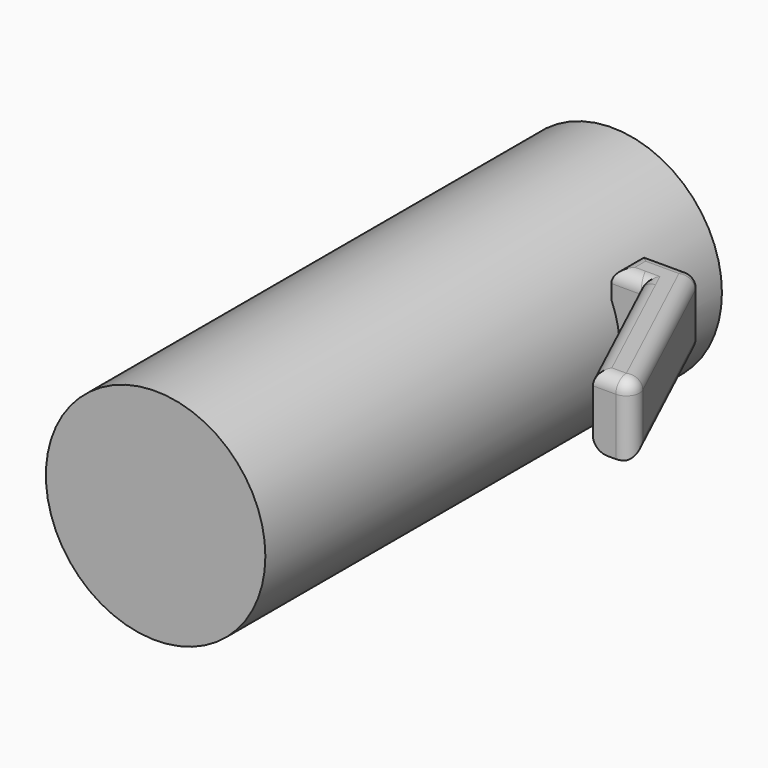
from build123d import *

# Parameters (mm, degrees)
F0_R          = 31.75
F0_R_2        = 28.575
F1_DEPTH      = 165.1
F3_DEPTH      = 20.32
F4_T1_DEPTH   = 16.51
F4_T3_DEPTH   = 12.7
F4_T5_DEPTH   = 50.1912424643
F4_T7_DEPTH   = 13.4477623063
F4_T9_DEPTH   = 11.43
F4_T14_DEPTH  = 3.8862
F4_T20_DEPTH  = 3.8862
F4_T26_DEPTH  = 3.8862
F4_T32_DEPTH  = 65.6967445131
F4_T37_DEPTH  = 18.118286919
F4_T42_DEPTH  = 65.037372593
F4_T48_DEPTH  = 16.1561075649
F4_T53_DEPTH  = 65.037372593
F4_T59_DEPTH  = 20.4327623063
F4_S60_R      = 31.75
F4_T61_DEPTH  = 12
F4_T66_DEPTH  = 65.6967445131
F4_T70_DEPTH  = 31.461255122
F4_T77_DEPTH  = 20.955
F4_T81_DEPTH  = 22.9727623063
F4_T88_DEPTH  = 27.643286919
F4_T92_DEPTH  = 20.955
F4_T99_DEPTH  = 18.118286919
F4_T103_DEPTH = 65.037372593
F4_T110_DEPTH = 16.1561075649
F4_T114_DEPTH = 65.037372593
F5_R          = 27.6352
F6_DEPTH      = 161.925


# Not quite as in the source:
# - a fillet or chamfer that OpenCascade refuses, or shapes differently, is made with other operations: its cross-section is extruded or revolved along the edge and cut away or added


with BuildPart() as f1:
    # F0 (on Front) → F1 (new body)
    with BuildSketch(Plane.XZ):
        Circle(F0_R)
        Circle(F0_R_2, mode=Mode.SUBTRACT)
        Circle(F0_R_2)
    extrude(amount=F1_DEPTH)

    # F2 (on Top) → F3 (join)
    with BuildSketch(Plane.XY):
        Polygon((45.085, -25.4), (29.21, -25.4), (29.21, -36.83), (37.803286919, -36.83), (57.2383903863, -78.5087138864), (69.85, -78.5087138864), align=None)
    extrude(amount=F3_DEPTH)

    # F4: fillet of radius 3.81 on 11 edges, made by hand

    # F4_s2 → F4_t1 (cut)
    with BuildSketch(Plane.XY):
        with BuildLine():
            ThreePointArc((67.3225306198, -73.0885383092), (67.0828193597, -76.7458253942), (63.8694979512, -78.5087138864))
            Line((63.8694979512, -78.5087138864), (63.8694979512, -78.5849138864))
            Line((63.8694979512, -78.5849138864), (69.969610041, -78.5849138864))
            Line((69.969610041, -78.5849138864), (67.3915912732, -73.0563347976))
            Line((67.3915912732, -73.0563347976), (67.3225306198, -73.0885383092))
        make_face()
    extrude(amount=F4_T1_DEPTH, mode=Mode.SUBTRACT)

    # F4_s4 → F4_t3 (cut)
    with BuildSketch(Plane.XY.offset(3.81)):
        with BuildLine():
            ThreePointArc((42.6577623063, -25.4), (44.7048738141, -25.9966785915), (46.1107949749, -27.5998244228))
            Line((46.1107949749, -27.5998244228), (46.1798556283, -27.5676209112))
            Line((46.1798556283, -27.5676209112), (45.1335447539, -25.3238))
            Line((45.1335447539, -25.3238), (42.6577623063, -25.3238))
            Line((42.6577623063, -25.3238), (42.6577623063, -25.4))
        make_face()
    extrude(amount=F4_T3_DEPTH, mode=Mode.SUBTRACT)

    # F4_s6 → F4_t5 (cut)
    with BuildSketch(Plane(origin=(40.018755356, -85.8204978112, 0), x_dir=(0, 0, 1), z_dir=(-0.4226182617, 0.906307787, 0))):
        with BuildLine():
            ThreePointArc((16.51, 30.1263827303), (19.2040768363, 29.0104595667), (20.32, 26.3163827303))
            Line((20.32, 26.3163827303), (20.3962, 26.3163827303))
            Line((20.3962, 26.3163827303), (20.3962, 30.2025827303))
            Line((20.3962, 30.2025827303), (16.51, 30.2025827303))
            Line((16.51, 30.2025827303), (16.51, 30.1263827303))
        make_face()
    extrude(amount=F4_T5_DEPTH, mode=Mode.SUBTRACT)

    # F4_s8 → F4_t7 (cut)
    with BuildSketch(Plane.YZ.offset(29.21)):
        with BuildLine():
            ThreePointArc((-25.4, 16.51), (-26.5159231637, 19.2040768363), (-29.21, 20.32))
            Line((-29.21, 20.32), (-29.21, 20.3962))
            Line((-29.21, 20.3962), (-25.3238, 20.3962))
            Line((-25.3238, 20.3962), (-25.3238, 16.51))
            Line((-25.3238, 16.51), (-25.4, 16.51))
        make_face()
    extrude(amount=F4_T7_DEPTH, mode=Mode.SUBTRACT)

    # F4_s10 → F4_t9 (cut)
    with BuildSketch(Plane.XZ.offset(25.4)):
        with BuildLine():
            ThreePointArc((29.21, 16.51), (30.3259231637, 19.2040768363), (33.02, 20.32))
            Line((33.02, 20.32), (33.02, 20.3962))
            Line((33.02, 20.3962), (29.1338, 20.3962))
            Line((29.1338, 20.3962), (29.1338, 16.51))
            Line((29.1338, 16.51), (29.21, 16.51))
        make_face()
    extrude(amount=F4_T9_DEPTH, mode=Mode.SUBTRACT)


with BuildPart() as f4_tool12:
    # F4_s13 → F4_t14 (new body)
    with BuildSketch(Plane.XY.offset(16.51)):
        Polygon((63.8694979512, -74.6987138864), (67.3915912732, -73.0563347976), (69.969610041, -78.5849138864), (63.8694979512, -78.5849138864), align=None)
    extrude(amount=F4_T14_DEPTH)

    # F4_s15 → F4_t16 (revolve, cut)
    with BuildSketch(Plane(origin=(63.8694979512, -74.6987138864, 16.51), x_dir=(-0.8433914458, 0.5372996083, 0), z_dir=(0.5372996083, 0.8433914458, 0))):
        with BuildLine():
            ThreePointArc((0, -3.81), (3.81, 0), (0, 3.81))
            Line((0, 3.81), (0, -3.81))
        make_face()
    revolve(axis=Axis((63.8694979512, -74.6987138864, 16.51), (0, 0, 1)), mode=Mode.SUBTRACT)


with BuildPart() as f1_1:
    add(f1.part)

    # F4_t11: cut F4_tool12
    add(f4_tool12.part, mode=Mode.SUBTRACT)


with BuildPart() as f4_tool18:
    # F4_s19 → F4_t20 (new body)
    with BuildSketch(Plane.XY.offset(3.81)):
        Polygon((42.6577623063, -29.21), (42.6577623063, -25.3238), (45.1335447539, -25.3238), (46.1798556283, -27.5676209112), align=None)
    extrude(amount=-F4_T20_DEPTH)

    # F4_s21 → F4_t22 (revolve, cut)
    with BuildSketch(Plane(origin=(42.6577623063, -29.21, 3.81), x_dir=(-0.5372996083, -0.8433914458, 0), z_dir=(0.8433914458, -0.5372996083, 0))):
        with BuildLine():
            ThreePointArc((0, -3.81), (3.81, 0), (0, 3.81))
            Line((0, 3.81), (0, -3.81))
        make_face()
    revolve(axis=Axis((42.6577623063, -29.21, 3.81), (0, 0, -1)), mode=Mode.SUBTRACT)


with BuildPart() as f1_2:
    add(f1_1.part)

    # F4_t17: cut F4_tool18
    add(f4_tool18.part, mode=Mode.SUBTRACT)


with BuildPart() as f4_tool24:
    # F4_s25 → F4_t26 (new body)
    with BuildSketch(Plane.XY.offset(16.51)):
        Polygon((42.6577623063, -29.21), (42.6577623063, -25.3238), (45.1335447539, -25.3238), (46.1798556283, -27.5676209112), align=None)
    extrude(amount=F4_T26_DEPTH)

    # F4_s27 → F4_t28 (revolve, cut)
    with BuildSketch(Plane(origin=(42.6577623063, -29.21, 16.51), x_dir=(-0.5372996083, -0.8433914458, 0), z_dir=(-0.8433914458, 0.5372996083, 0))):
        with BuildLine():
            ThreePointArc((0, -3.81), (3.81, 0), (0, 3.81))
            Line((0, 3.81), (0, -3.81))
        make_face()
    revolve(axis=Axis((42.6577623063, -29.21, 16.51), (0, 0, 1)), mode=Mode.SUBTRACT)


with BuildPart() as f1_3:
    add(f1_2.part)

    # F4_t23: cut F4_tool24
    add(f4_tool24.part, mode=Mode.SUBTRACT)


with BuildPart() as f4_tool30:
    # F4_s31 → F4_t32 (new body)
    with BuildSketch(Plane(origin=(46.5716636793, -99.87325506, 0), x_dir=(0, 0, 1), z_dir=(-0.4226182617, 0.906307787, 0))):
        with BuildLine():
            ThreePointArc((0, 26.3163827303), (1.1159231637, 29.0104595667), (3.81, 30.1263827303))
            Line((3.81, 30.1263827303), (3.81, 30.2025827303))
            Line((3.81, 30.2025827303), (-0.0762, 30.2025827303))
            Line((-0.0762, 30.2025827303), (-0.0762, 26.3163827303))
            Line((-0.0762, 26.3163827303), (0, 26.3163827303))
        make_face()
    extrude(amount=F4_T32_DEPTH)

    split(bisect_by=Plane.XZ.offset(78.5087138864), keep=Keep.BOTTOM)


with BuildPart() as f1_4:
    add(f1_3.part)

    # F4_t29: cut F4_tool30
    add(f4_tool30.part, mode=Mode.SUBTRACT)


with BuildPart() as f4_tool35:
    # F4_s36 → F4_t37 (new body)
    with BuildSketch(Plane.YZ.offset(29.21)):
        with BuildLine():
            ThreePointArc((-36.83, 16.51), (-35.7140768363, 19.2040768363), (-33.02, 20.32))
            Line((-33.02, 20.32), (-33.02, 20.3962))
            Line((-33.02, 20.3962), (-36.9062, 20.3962))
            Line((-36.9062, 20.3962), (-36.9062, 16.51))
            Line((-36.9062, 16.51), (-36.83, 16.51))
        make_face()
    extrude(amount=F4_T37_DEPTH)

    split(bisect_by=Plane(origin=(16.9446772579, 7.9014327703, 0), x_dir=(0, 0, 1), z_dir=(-0.906307787, -0.4226182617, 0)), keep=Keep.TOP)


with BuildPart() as f1_5:
    add(f1_4.part)

    # F4_t34: cut F4_tool35
    add(f4_tool35.part, mode=Mode.SUBTRACT)


with BuildPart() as f4_tool40:
    # F4_s41 → F4_t42 (new body)
    with BuildSketch(Plane(origin=(16.833170718, -36.0988510988, 0), x_dir=(0, 0, 1), z_dir=(0.4226182617, -0.906307787, 0))):
        with BuildLine():
            ThreePointArc((16.51, -18.6963827303), (19.2040768363, -19.812305894), (20.32, -22.5063827303))
            Line((20.32, -22.5063827303), (20.3962, -22.5063827303))
            Line((20.3962, -22.5063827303), (20.3962, -18.6201827303))
            Line((20.3962, -18.6201827303), (16.51, -18.6201827303))
            Line((16.51, -18.6201827303), (16.51, -18.6963827303))
        make_face()
    extrude(amount=F4_T42_DEPTH)

    split(bisect_by=Plane.XZ.offset(36.83), keep=Keep.TOP)

    split(bisect_by=Plane.XZ.offset(78.5087138864), keep=Keep.BOTTOM)


with BuildPart() as f1_6:
    add(f1_5.part)

    # F4_t39: cut F4_tool40
    add(f4_tool40.part, mode=Mode.SUBTRACT)


with BuildPart() as f4_tool46:
    # F4_s47 → F4_t48 (new body)
    with BuildSketch(Plane.YZ.offset(47.7133903863)):
        with BuildLine():
            ThreePointArc((-78.5087138864, 16.51), (-77.3927907227, 19.2040768363), (-74.6987138864, 20.32))
            Line((-74.6987138864, 20.32), (-74.6987138864, 20.3962))
            Line((-74.6987138864, 20.3962), (-78.5849138864, 20.3962))
            Line((-78.5849138864, 20.3962), (-78.5849138864, 16.51))
            Line((-78.5849138864, 16.51), (-78.5087138864, 16.51))
        make_face()
    extrude(amount=F4_T48_DEPTH)

    split(bisect_by=Plane(origin=(16.9446772579, 7.9014327703, 0), x_dir=(0, 0, 1), z_dir=(0.906307787, 0.4226182617, 0)), keep=Keep.TOP)


with BuildPart() as f1_7:
    add(f1_6.part)

    # F4_t45: cut F4_tool46
    add(f4_tool46.part, mode=Mode.SUBTRACT)


with BuildPart() as f4_tool51:
    # F4_s52 → F4_t53 (new body)
    with BuildSketch(Plane(origin=(16.833170718, -36.0988510988, 0), x_dir=(0, 0, 1), z_dir=(0.4226182617, -0.906307787, 0))):
        with BuildLine():
            ThreePointArc((0, -22.5063827303), (1.1159231637, -19.812305894), (3.81, -18.6963827303))
            Line((3.81, -18.6963827303), (3.81, -18.6201827303))
            Line((3.81, -18.6201827303), (-0.0762, -18.6201827303))
            Line((-0.0762, -18.6201827303), (-0.0762, -22.5063827303))
            Line((-0.0762, -22.5063827303), (0, -22.5063827303))
        make_face()
    extrude(amount=F4_T53_DEPTH)

    split(bisect_by=Plane.XZ.offset(78.5087138864), keep=Keep.BOTTOM)

    split(bisect_by=Plane.XZ.offset(36.83), keep=Keep.TOP)


with BuildPart() as f1_8:
    add(f1_7.part)

    # F4_t50: cut F4_tool51
    add(f4_tool51.part, mode=Mode.SUBTRACT)


with BuildPart() as f4_tool57:
    # F4_s58 → F4_t59 (new body)
    with BuildSketch(Plane.YZ.offset(42.6577623063)):
        with BuildLine():
            ThreePointArc((-29.21, 0), (-26.5159231637, 1.1159231637), (-25.4, 3.81))
            Line((-25.4, 3.81), (-25.3238, 3.81))
            Line((-25.3238, 3.81), (-25.3238, -0.0762))
            Line((-25.3238, -0.0762), (-29.21, -0.0762))
            Line((-29.21, -0.0762), (-29.21, 0))
        make_face()
    extrude(amount=-F4_T59_DEPTH)

    # F4_s60 → F4_t61 (cut, symmetric)
    with BuildSketch(Plane.XZ.offset(27.3)):
        Circle(F4_S60_R)
    extrude(amount=F4_T61_DEPTH, both=True, mode=Mode.SUBTRACT)


with BuildPart() as f1_9:
    add(f1_8.part)

    # F4_t56: cut F4_tool57
    add(f4_tool57.part, mode=Mode.SUBTRACT)


with BuildPart() as f4_tool64:
    # F4_s65 → F4_t66 (new body)
    with BuildSketch(Plane(origin=(46.5716636793, -99.87325506, 0), x_dir=(0, 0, 1), z_dir=(-0.4226182617, 0.906307787, 0))):
        with BuildLine():
            ThreePointArc((0, 26.3163827303), (1.1159231637, 29.0104595667), (3.81, 30.1263827303))
            Line((3.81, 30.1263827303), (3.81, 30.2025827303))
            Line((3.81, 30.2025827303), (-0.0762, 30.2025827303))
            Line((-0.0762, 30.2025827303), (-0.0762, 26.3163827303))
            Line((-0.0762, 26.3163827303), (0, 26.3163827303))
        make_face()
    extrude(amount=F4_T66_DEPTH)

    split(bisect_by=Plane.XZ.offset(78.5087138864), keep=Keep.TOP)


with BuildPart() as f4_tool68:
    # F4_s69 → F4_t70 (new body)
    with BuildSketch(Plane.XY.offset(-14.951255122)):
        with BuildLine():
            ThreePointArc((67.3225306198, -73.0885383092), (67.0828193597, -76.7458253942), (63.8694979512, -78.5087138864))
            Line((63.8694979512, -78.5087138864), (63.8694979512, -78.5849138864))
            Line((63.8694979512, -78.5849138864), (69.969610041, -78.5849138864))
            Line((69.969610041, -78.5849138864), (67.3915912732, -73.0563347976))
            Line((67.3915912732, -73.0563347976), (67.3225306198, -73.0885383092))
        make_face()
    extrude(amount=F4_T70_DEPTH)

    split(bisect_by=Plane.XY, keep=Keep.BOTTOM)


with BuildPart() as f4_tool64_1:
    add(f4_tool64.part)

    # F4_t72: intersect F4_tool68
    add(f4_tool68.part, mode=Mode.INTERSECT)


with BuildPart() as f1_10:
    add(f1_9.part)

    # F4_t62: cut F4_tool64
    add(f4_tool64_1.part, mode=Mode.SUBTRACT)


with BuildPart() as f4_tool75:
    # F4_s76 → F4_t77 (new body)
    with BuildSketch(Plane.XZ.offset(15.875)):
        with BuildLine():
            ThreePointArc((29.21, 16.51), (30.3259231637, 19.2040768363), (33.02, 20.32))
            Line((33.02, 20.32), (33.02, 20.3962))
            Line((33.02, 20.3962), (29.1338, 20.3962))
            Line((29.1338, 20.3962), (29.1338, 16.51))
            Line((29.1338, 16.51), (29.21, 16.51))
        make_face()
    extrude(amount=F4_T77_DEPTH)

    split(bisect_by=Plane.XZ.offset(25.4), keep=Keep.BOTTOM)


with BuildPart() as f4_tool79:
    # F4_s80 → F4_t81 (new body)
    with BuildSketch(Plane.YZ.offset(42.6577623063)):
        with BuildLine():
            ThreePointArc((-25.4, 16.51), (-26.5159231637, 19.2040768363), (-29.21, 20.32))
            Line((-29.21, 20.32), (-29.21, 20.3962))
            Line((-29.21, 20.3962), (-25.3238, 20.3962))
            Line((-25.3238, 20.3962), (-25.3238, 16.51))
            Line((-25.3238, 16.51), (-25.4, 16.51))
        make_face()
    extrude(amount=-F4_T81_DEPTH)

    split(bisect_by=Plane.YZ.offset(29.21), keep=Keep.BOTTOM)


with BuildPart() as f4_tool75_1:
    add(f4_tool75.part)

    # F4_t83: intersect F4_tool79
    add(f4_tool79.part, mode=Mode.INTERSECT)


with BuildPart() as f1_11:
    add(f1_10.part)

    # F4_t73: cut F4_tool75
    add(f4_tool75_1.part, mode=Mode.SUBTRACT)


with BuildPart() as f4_tool86:
    # F4_s87 → F4_t88 (new body)
    with BuildSketch(Plane.YZ.offset(19.685)):
        with BuildLine():
            ThreePointArc((-36.83, 16.51), (-35.7140768363, 19.2040768363), (-33.02, 20.32))
            Line((-33.02, 20.32), (-33.02, 20.3962))
            Line((-33.02, 20.3962), (-36.9062, 20.3962))
            Line((-36.9062, 20.3962), (-36.9062, 16.51))
            Line((-36.9062, 16.51), (-36.83, 16.51))
        make_face()
    extrude(amount=F4_T88_DEPTH)

    split(bisect_by=Plane.YZ.offset(29.21), keep=Keep.BOTTOM)


with BuildPart() as f4_tool90:
    # F4_s91 → F4_t92 (new body)
    with BuildSketch(Plane.XZ.offset(25.4)):
        with BuildLine():
            ThreePointArc((29.21, 16.51), (30.3259231637, 19.2040768363), (33.02, 20.32))
            Line((33.02, 20.32), (33.02, 20.3962))
            Line((33.02, 20.3962), (29.1338, 20.3962))
            Line((29.1338, 20.3962), (29.1338, 16.51))
            Line((29.1338, 16.51), (29.21, 16.51))
        make_face()
    extrude(amount=F4_T92_DEPTH)

    split(bisect_by=Plane.XZ.offset(36.83), keep=Keep.TOP)


with BuildPart() as f4_tool86_1:
    add(f4_tool86.part)

    # F4_t94: intersect F4_tool90
    add(f4_tool90.part, mode=Mode.INTERSECT)


with BuildPart() as f1_12:
    add(f1_11.part)

    # F4_t84: cut F4_tool86
    add(f4_tool86_1.part, mode=Mode.SUBTRACT)


with BuildPart() as f4_tool97:
    # F4_s98 → F4_t99 (new body)
    with BuildSketch(Plane.YZ.offset(29.21)):
        with BuildLine():
            ThreePointArc((-36.83, 16.51), (-35.7140768363, 19.2040768363), (-33.02, 20.32))
            Line((-33.02, 20.32), (-33.02, 20.3962))
            Line((-33.02, 20.3962), (-36.9062, 20.3962))
            Line((-36.9062, 20.3962), (-36.9062, 16.51))
            Line((-36.9062, 16.51), (-36.83, 16.51))
        make_face()
    extrude(amount=F4_T99_DEPTH)

    split(bisect_by=Plane(origin=(16.9446772579, 7.9014327703, 0), x_dir=(0, 0, 1), z_dir=(0.906307787, 0.4226182617, 0)), keep=Keep.TOP)


with BuildPart() as f4_tool101:
    # F4_s102 → F4_t103 (new body)
    with BuildSketch(Plane(origin=(16.833170718, -36.0988510988, 0), x_dir=(0, 0, 1), z_dir=(0.4226182617, -0.906307787, 0))):
        with BuildLine():
            ThreePointArc((16.51, -18.6963827303), (19.2040768363, -19.812305894), (20.32, -22.5063827303))
            Line((20.32, -22.5063827303), (20.3962, -22.5063827303))
            Line((20.3962, -22.5063827303), (20.3962, -18.6201827303))
            Line((20.3962, -18.6201827303), (16.51, -18.6201827303))
            Line((16.51, -18.6201827303), (16.51, -18.6963827303))
        make_face()
    extrude(amount=F4_T103_DEPTH)

    split(bisect_by=Plane.XZ.offset(36.83), keep=Keep.BOTTOM)


with BuildPart() as f4_tool97_1:
    add(f4_tool97.part)

    # F4_t105: intersect F4_tool101
    add(f4_tool101.part, mode=Mode.INTERSECT)


with BuildPart() as f1_13:
    add(f1_12.part)

    # F4_t95: cut F4_tool97
    add(f4_tool97_1.part, mode=Mode.SUBTRACT)


with BuildPart() as f4_tool108:
    # F4_s109 → F4_t110 (new body)
    with BuildSketch(Plane.YZ.offset(47.7133903863)):
        with BuildLine():
            ThreePointArc((-78.5087138864, 16.51), (-77.3927907227, 19.2040768363), (-74.6987138864, 20.32))
            Line((-74.6987138864, 20.32), (-74.6987138864, 20.3962))
            Line((-74.6987138864, 20.3962), (-78.5849138864, 20.3962))
            Line((-78.5849138864, 20.3962), (-78.5849138864, 16.51))
            Line((-78.5849138864, 16.51), (-78.5087138864, 16.51))
        make_face()
    extrude(amount=F4_T110_DEPTH)

    split(bisect_by=Plane(origin=(16.9446772579, 7.9014327703, 0), x_dir=(0, 0, 1), z_dir=(-0.906307787, -0.4226182617, 0)), keep=Keep.TOP)


with BuildPart() as f4_tool112:
    # F4_s113 → F4_t114 (new body)
    with BuildSketch(Plane(origin=(16.833170718, -36.0988510988, 0), x_dir=(0, 0, 1), z_dir=(0.4226182617, -0.906307787, 0))):
        with BuildLine():
            ThreePointArc((16.51, -18.6963827303), (19.2040768363, -19.812305894), (20.32, -22.5063827303))
            Line((20.32, -22.5063827303), (20.3962, -22.5063827303))
            Line((20.3962, -22.5063827303), (20.3962, -18.6201827303))
            Line((20.3962, -18.6201827303), (16.51, -18.6201827303))
            Line((16.51, -18.6201827303), (16.51, -18.6963827303))
        make_face()
    extrude(amount=F4_T114_DEPTH)

    split(bisect_by=Plane.XZ.offset(78.5087138864), keep=Keep.TOP)


with BuildPart() as f4_tool108_1:
    add(f4_tool108.part)

    # F4_t116: intersect F4_tool112
    add(f4_tool112.part, mode=Mode.INTERSECT)


with BuildPart() as f1_14:
    add(f1_13.part)

    # F4_t106: cut F4_tool108
    add(f4_tool108_1.part, mode=Mode.SUBTRACT)

    # F5 (on face) → F6 (cut)
    with BuildSketch(Plane(origin=(0, 0, 0), x_dir=(-1, 0, 0), z_dir=(0, 1, 0))):
        Circle(F5_R)
    extrude(amount=-F6_DEPTH, mode=Mode.SUBTRACT)


solid = f1_14.part
